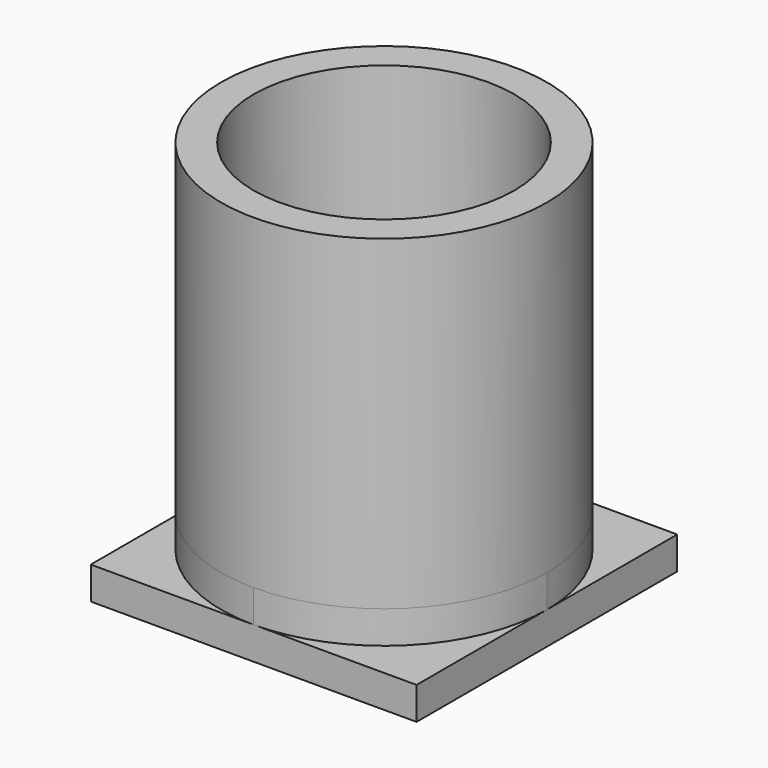
from build123d import *

# Parameters (mm, degrees)
F0_R     = 0.635
F1_DEPTH = 1.27
F2_R     = 0.508
F3_DEPTH = 1.016
F5_DEPTH = 0.254
F6_DEPTH = 0.127
F7_R     = 0.1016
F8_DEPTH = 25.4


with BuildPart() as f1:
    # F0 (on Top) → F1 (new body)
    with BuildSketch(Plane.XY):
        Circle(F0_R)
    extrude(amount=F1_DEPTH)

    # F2 (on face) → F3 (cut)
    with BuildSketch(Plane.XY.offset(1.27)):
        Circle(F2_R)
    extrude(amount=-F3_DEPTH, mode=Mode.SUBTRACT)

    # F4 (on face) → F5 (join)
    with BuildSketch(Plane(origin=(0, 0, 0), x_dir=(1, 0, 0), z_dir=(0, 0, -1))):
        with BuildLine():
            Line((0.635, 0), (0.635, 0.635))
            Line((0.635, 0.635), (0, 0.635))
            ThreePointArc((0, 0.635), (0.4490128061, 0.4490128061), (0.635, 0))
        make_face()
        with BuildLine():
            ThreePointArc((-0.635, 0), (-0.4490128061, 0.4490128061), (0, 0.635))
            Line((0, 0.635), (-0.635, 0.635))
            Line((-0.635, 0.635), (-0.635, 0))
        make_face()
        with BuildLine():
            ThreePointArc((0.635, 0), (0.4490128061, 0.4490128061), (0, 0.635))
            ThreePointArc((0, 0.635), (-0.4490128061, 0.4490128061), (-0.635, 0))
            ThreePointArc((-0.635, 0), (-0.4490128061, -0.4490128061), (0, -0.635))
            ThreePointArc((0, -0.635), (0.4490128061, -0.4490128061), (0.635, 0))
        make_face()
        with BuildLine():
            Line((0.635, -0.635), (0.635, 0))
            ThreePointArc((0.635, 0), (0.4490128061, -0.4490128061), (0, -0.635))
            Line((0, -0.635), (0.635, -0.635))
        make_face()
        with BuildLine():
            ThreePointArc((0, -0.635), (-0.4490128061, -0.4490128061), (-0.635, 0))
            Line((-0.635, 0), (-0.635, -0.635))
            Line((-0.635, -0.635), (0, -0.635))
        make_face()
    extrude(amount=F5_DEPTH)

    # F6 (cut): faces of the model
    f6_faces = [f1.faces().sort_by_distance(p)[0] for p in [
        (-0.4931613588, 0.4931613588, 0),
        (-0.4931613588, -0.4931613588, 0),
        (0.4931613588, -0.4931613588, 0),
        (0.4931613588, 0.4931613588, 0),
    ]]
    extrude(f6_faces, amount=-F6_DEPTH, mode=Mode.SUBTRACT)

    # F7 (on face) → F8 (cut)
    with BuildSketch(Plane(origin=(0, 0, -0.254), x_dir=(1, 0, 0), z_dir=(0, 0, -1))):
        Circle(F7_R)
    extrude(amount=-F8_DEPTH, mode=Mode.SUBTRACT)


solid = f1.part
